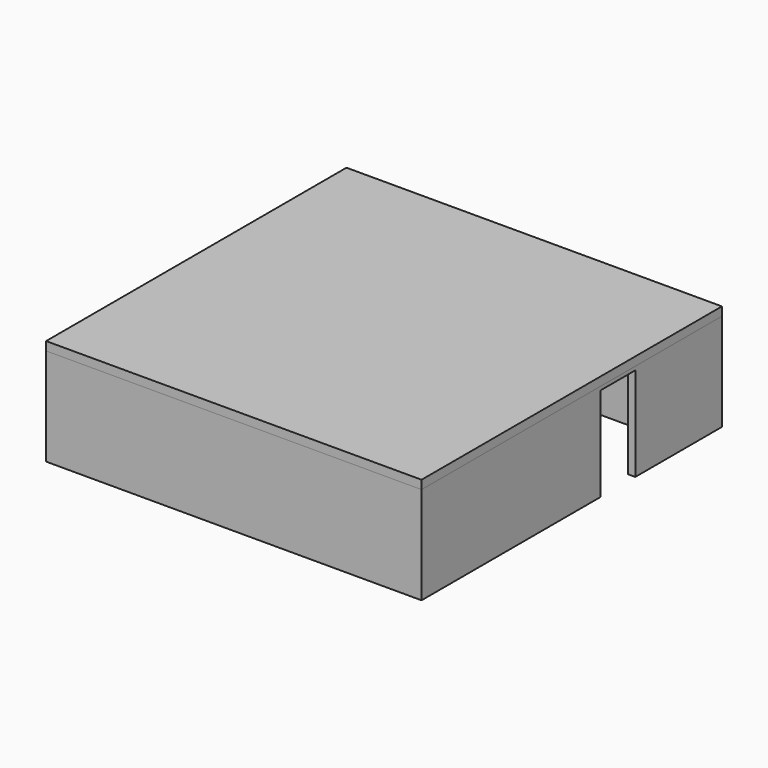
from build123d import *

# Parameters (mm, degrees)
F0_W      = 660.4
F0_H      = 660.4
F1_DEPTH  = 171.45
F3_W      = 635
F3_H      = 635
F4_DEPTH  = 251.46
F5_W      = 76.2
F5_H      = 165.1
F6_DEPTH  = 12.7
F7_W      = 635
F7_H      = 10.16
F8_DEPTH  = 171.45
F9_W      = 254
F9_H      = 171.45
F10_DEPTH = 10.16
F11_W     = 660.4
F11_H     = 660.4
F12_DEPTH = 15.24
F14_DEPTH = 76.2
F15_W     = 76.2
F15_H     = 152.4
F16_DEPTH = 10.16
F17_W     = 10.16
F17_H     = 171.45
F18_DEPTH = 330.2
F20_DEPTH = 76.2
F21_W     = 63.5
F21_H     = 63.5
F22_DEPTH = 160.528
F23_W     = 10.16
F23_H     = 330.2
F24_DEPTH = 171.45
F25_W     = 177.385084331
F25_H     = 54.4112967327
F26_DEPTH = 7.62


with BuildPart() as f1:
    # F0 (on Top) → F1 (new body)
    with BuildSketch(Plane.XY):
        Rectangle(F0_W, F0_H)
    extrude(amount=F1_DEPTH)

    # F3 (on face) → F4 (cut)
    with BuildSketch(Plane.XY.offset(171.45)):
        Rectangle(F3_W, F3_H)
    extrude(amount=-F4_DEPTH, mode=Mode.SUBTRACT)

    # F5 (on face) → F6 (cut, through all)
    with BuildSketch(Plane.YZ.offset(330.2)):
        with Locations((101.6, 82.55)):
            Rectangle(F5_W, F5_H)
    extrude(amount=-F6_DEPTH, mode=Mode.SUBTRACT)

    # F7 (on face) → F8 (join, through all)
    with BuildSketch(Plane.XY):
        with Locations((0, -17.78)):
            Rectangle(F7_W, F7_H)
    extrude(amount=F8_DEPTH)

    # F9 (on face) → F10 (cut, through all)
    with BuildSketch(Plane.XZ.offset(22.86)):
        with Locations((190.5, 85.725)):
            Rectangle(F9_W, F9_H)
    extrude(amount=-F10_DEPTH, mode=Mode.SUBTRACT)

    # F15 (on face) → F16 (cut, through all)
    with BuildSketch(Plane.XZ.offset(22.86)):
        with Locations((-61.403836852, 76.2)):
            Rectangle(F15_W, F15_H)
    extrude(amount=-F16_DEPTH, mode=Mode.SUBTRACT)

    # F17 (on face) → F18 (join, through all)
    with BuildSketch(Plane(origin=(0, -12.7, 0), x_dir=(-1, 0, 0), z_dir=(0, 1, 0))):
        with Locations((-58.42, 85.725)):
            Rectangle(F17_W, F17_H)
    extrude(amount=F18_DEPTH)

    # F23 (on face) → F24 (join, through all)
    with BuildSketch(Plane.XY):
        with Locations((-127.1187807751, 152.4)):
            Rectangle(F23_W, F23_H)
    extrude(amount=F24_DEPTH)


with BuildPart() as f12:
    # F11 (on face) → F12 (new body)
    with BuildSketch(Plane.XY.offset(171.45)):
        Rectangle(F11_W, F11_H)
    extrude(amount=F12_DEPTH)


with BuildPart() as f14:
    # F13 (on face) → F14 (new body)
    with BuildSketch(Plane.XY):
        with BuildLine():
            Line((5.9782206564, 300.767604221), (-64.3982206564, 300.767604221))
            ThreePointArc((-64.3982206564, 300.767604221), (-86.36, 278.8058248774), (-64.3982206564, 256.8440455338))
            Line((-64.3982206564, 256.8440455338), (5.9782206564, 256.8440455338))
            ThreePointArc((5.9782206564, 256.8440455338), (27.94, 278.8058248774), (5.9782206564, 300.767604221))
        make_face()
    extrude(amount=F14_DEPTH)


with BuildPart() as f14b:
    # F13 (on face) → F14, piece 2 (new body)
    with BuildSketch(Plane.XY):
        Polygon((27.94, 200.0615537474), (27.94, 230.4656018443), (7.62, 230.4656018443), (7.62, 225.4574813614), (7.62, 203.4733542914), (7.62, 200.0615537474), align=None)
        with BuildLine():
            Line((7.62, 203.4733542914), (7.62, 225.4574813614))
            Line((7.62, 225.4574813614), (-3.372063535, 225.4574813614))
            ThreePointArc((-3.372063535, 225.4574813614), (-14.36412707, 214.4654178264), (-3.372063535, 203.4733542914))
            Line((-3.372063535, 203.4733542914), (7.62, 203.4733542914))
        make_face()
    extrude(amount=F14_DEPTH)


with BuildPart() as f20:
    # F19 (on face) → F20 (new body)
    with BuildSketch(Plane.XY):
        Polygon((127, 317.5), (63.5, 317.5), (63.5, 254), (63.5, 41.0446626544), (63.5, -22.4553373456), (127, -22.4553373456), (240.885084331, -22.4553373456), (240.885084331, 41.0446626544), (127, 41.0446626544), (127, 254), (242.7029758692, 254), (242.7029758692, 317.5), align=None)
    extrude(amount=F20_DEPTH)

    # F25 (on face) → F26 (join)
    with BuildSketch(Plane.XY.offset(76.2)):
        with Locations((152.1925421655, -21.7650732957)):
            Rectangle(F25_W, F25_H)
    extrude(amount=-F26_DEPTH)


with BuildPart() as f22:
    # F21 (on face) → F22 (new body)
    with BuildSketch(Plane.XY):
        with Locations((280.3060774803, 282.0997173786)):
            Rectangle(F21_W, F21_H)
    extrude(amount=F22_DEPTH)


solid = Compound([f1.part, f12.part, f14.part, f14b.part, f20.part, f22.part])
